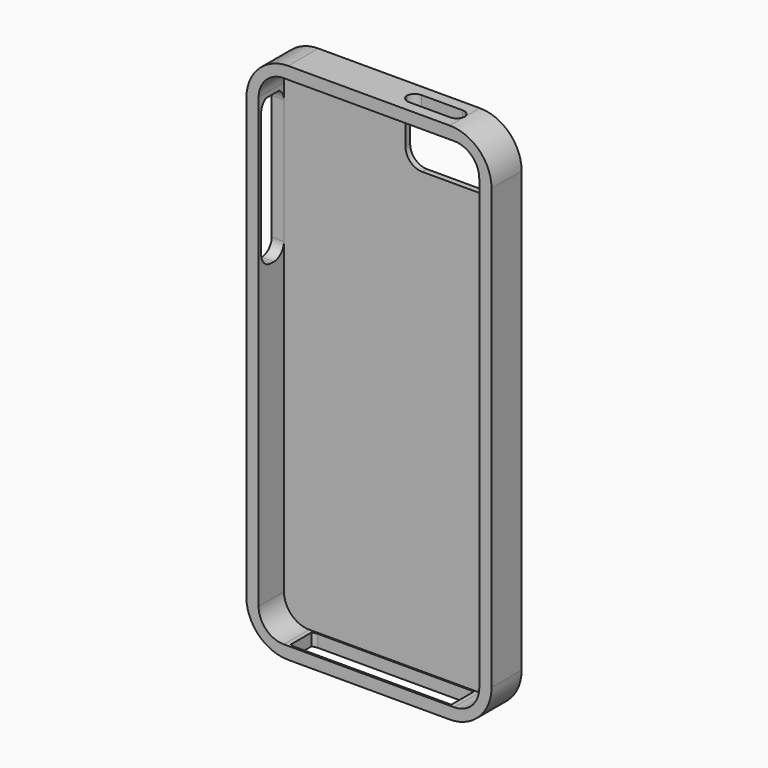
from build123d import *

# Parameters (mm, degrees)
F1_DEPTH      = 9
F3_DEPTH      = 5
F5_DEPTH      = 5.53
F7_DEPTH      = 7.6
F9_DEPTH      = 3
F11_DEPTH     = 25
F12_DEPTH     = 25
F14_DEPTH     = 8
F15_T         = 2.5
F15_T3_DEPTH  = 7.928932
F15_T5_DEPTH  = 13
F15_T7_DEPTH  = 45.742136
F15_T9_DEPTH  = 112.142136
F15_T11_DEPTH = 7.928932
F15_T13_DEPTH = 7.928932
F15_T16_ANGLE = 90
F15_T18_ANGLE = 90
F15_T20_ANGLE = 90
F15_T22_ANGLE = 90


# Not quite as in the source:
# - a shell that OpenCascade refuses in one call is made with other operations: the cavity is built on its own and cut out


with BuildPart() as f1:
    # F0 (on Front) → F1 (new body)
    with BuildSketch(Plane.XZ):
        with BuildLine():
            Line((13.970302, 55.774098), (-24.629698, 55.774098))
            ThreePointArc((-24.629698, 55.774098), (-31.700766, 52.845166), (-34.629698, 45.774098))
            Line((-34.629698, 45.774098), (-34.629698, -59.225902))
            ThreePointArc((-34.629698, -59.225902), (-31.700766, -66.29697), (-24.629698, -69.225902))
            Line((-24.629698, -69.225902), (13.970302, -69.225902))
            ThreePointArc((13.970302, -69.225902), (21.04137, -66.29697), (23.970302, -59.225902))
            Line((23.970302, -59.225902), (23.970302, 45.774098))
            ThreePointArc((23.970302, 45.774098), (21.04137, 52.845166), (13.970302, 55.774098))
        make_face()
    extrude(amount=F1_DEPTH)

    # F2 (on face) → F3 (cut)
    with BuildSketch(Plane(origin=(-34.629698, 0, 0), x_dir=(0, -1, 0), z_dir=(-1, 0, 0))):
        with BuildLine():
            ThreePointArc((1.445644, 13.40758), (2.324323, 11.28626), (4.445644, 10.40758))
            Line((4.445644, 10.40758), (5.235644, 10.40758))
            ThreePointArc((5.235644, 10.40758), (7.356964, 11.28626), (8.235644, 13.40758))
            Line((8.235644, 13.40758), (8.235644, 43.24758))
            ThreePointArc((8.235644, 43.24758), (7.867456, 44.687568), (6.853267, 45.774098))
            Line((6.853267, 45.774098), (2.82802, 45.774098))
            ThreePointArc((2.82802, 45.774098), (1.813831, 44.687568), (1.445644, 43.24758))
            Line((1.445644, 43.24758), (1.445644, 13.40758))
        make_face()
    extrude(amount=-F3_DEPTH, mode=Mode.SUBTRACT)

    # F4 (on face) → F5 (cut)
    with BuildSketch(Plane(origin=(0, 0, -69.225902), x_dir=(1, 0, 0), z_dir=(0, 0, -1))):
        with BuildLine():
            Line((13.596659, 8.527939), (-23.283341, 8.527939))
            ThreePointArc((-23.283341, 8.527939), (-23.975167, 8.447079), (-24.629698, 8.208858))
            Line((-24.629698, 8.208858), (-24.629698, 2.057021))
            ThreePointArc((-24.629698, 2.057021), (-23.975167, 1.818799), (-23.283341, 1.737939))
            Line((-23.283341, 1.737939), (13.596659, 1.737939))
            ThreePointArc((13.596659, 1.737939), (13.783845, 1.743785), (13.970302, 1.761298))
            Line((13.970302, 1.761298), (13.970302, 8.50458))
            ThreePointArc((13.970302, 8.50458), (13.783845, 8.522094), (13.596659, 8.527939))
        make_face()
    extrude(amount=-F5_DEPTH, mode=Mode.SUBTRACT)

    # F6 (on face) → F7 (cut)
    with BuildSketch(Plane.XZ.offset(9)):
        with BuildLine():
            Line((15.04137, 52.845166), (-25.700766, 52.845166))
            ThreePointArc((-25.700766, 52.845166), (-29.943407, 51.087807), (-31.700766, 46.845166))
            Line((-31.700766, 46.845166), (-31.700766, -60.29697))
            ThreePointArc((-31.700766, -60.29697), (-29.943407, -64.53961), (-25.700766, -66.29697))
            Line((-25.700766, -66.29697), (15.04137, -66.29697))
            ThreePointArc((15.04137, -66.29697), (19.28401, -64.53961), (21.04137, -60.29697))
            Line((21.04137, -60.29697), (21.04137, 46.845166))
            ThreePointArc((21.04137, 46.845166), (19.28401, 51.087807), (15.04137, 52.845166))
        make_face()
    extrude(amount=-F7_DEPTH, mode=Mode.SUBTRACT)

    # F8 (on face) → F9 (cut)
    with BuildSketch(Plane.XY.offset(55.774098)):
        with BuildLine():
            Line((2.150302, -6.363066), (11.970302, -6.363066))
            ThreePointArc((11.970302, -6.363066), (13.328609, -5.831058), (13.964286, -4.518066))
            ThreePointArc((13.964286, -4.518066), (13.328609, -3.205074), (11.970302, -2.673066))
            Line((11.970302, -2.673066), (2.150302, -2.673066))
            ThreePointArc((2.150302, -2.673066), (0.791994, -3.205074), (0.156317, -4.518066))
            ThreePointArc((0.156317, -4.518066), (0.791994, -5.831058), (2.150302, -6.363066))
        make_face()
    extrude(amount=-F9_DEPTH, mode=Mode.SUBTRACT)

    # F10 (on face) → F11 (cut)
    with BuildSketch(Plane(origin=(0, 0, 0), x_dir=(-1, 0, 0), z_dir=(0, 1, 0))):
        with BuildLine():
            Line((-1.330302, 51.964098), (-14.630302, 51.964098))
            ThreePointArc((-14.630302, 51.964098), (-17.458729, 50.792525), (-18.630302, 47.964098))
            Line((-18.630302, 47.964098), (-18.630302, 42.834098))
            ThreePointArc((-18.630302, 42.834098), (-17.458729, 40.005671), (-14.630302, 38.834098))
            Line((-14.630302, 38.834098), (-1.330302, 38.834098))
            ThreePointArc((-1.330302, 38.834098), (1.498125, 40.005671), (2.669698, 42.834098))
            Line((2.669698, 42.834098), (2.669698, 47.964098))
            ThreePointArc((2.669698, 47.964098), (1.498125, 50.792525), (-1.330302, 51.964098))
        make_face()
    extrude(amount=-F11_DEPTH, mode=Mode.SUBTRACT)

    # F4 (on face) → F12 (cut)
    with BuildSketch(Plane(origin=(0, 0, -69.225902), x_dir=(1, 0, 0), z_dir=(0, 0, -1))):
        with BuildLine():
            Line((13.596659, 8.527939), (-23.283341, 8.527939))
            ThreePointArc((-23.283341, 8.527939), (-23.975167, 8.447079), (-24.629698, 8.208858))
            Line((-24.629698, 8.208858), (-24.629698, 2.057021))
            ThreePointArc((-24.629698, 2.057021), (-23.975167, 1.818799), (-23.283341, 1.737939))
            Line((-23.283341, 1.737939), (13.596659, 1.737939))
            ThreePointArc((13.596659, 1.737939), (13.783845, 1.743785), (13.970302, 1.761298))
            Line((13.970302, 1.761298), (13.970302, 8.50458))
            ThreePointArc((13.970302, 8.50458), (13.783845, 8.522094), (13.596659, 8.527939))
        make_face()
    extrude(amount=-F12_DEPTH, mode=Mode.SUBTRACT)

    # F13 (on face) → F14 (join)
    with BuildSketch(Plane(origin=(0, 0, 0), x_dir=(-1, 0, 0), z_dir=(0, 1, 0))):
        Polygon((16.75532, 12.947292), (-7.00677, 12.947292), (-15.132455, 0), (-7.00677, 0), (-15.132455, -13.861218), (-7.00677, -13.861218), (-15.132455, -39.359054), (15.536753, -13.861218), (3.046423, -13.861218), (16.75532, 0), (6.702128, 0), align=None)
    extrude(amount=F14_DEPTH)

    # F15: shell of thickness 2.5, made by hand


with BuildPart() as f15_core1:
    # F15_t2: copy of F1
    add(f1.part)

    # the walls: a layer under each face that stays
    f15_faces = [f15_core1.faces().sort_by_distance(p)[0] for p in [
        (21.04137, -4.5, 52.845166),
        (23.970302, -4.5, -6.725902),
        (-5.329698, -4.5, 55.774098),
        (-32.676365, -9, -65.059235),
        (0.791994, -3.205074, 54.309632),
        (7.060302, -2.673066, 54.309632),
        (13.328609, -3.205074, 54.309632),
        (13.328609, -5.831058, 54.309632),
        (7.060302, -6.363066, 54.309632),
        (0.791994, -5.831058, 54.309632),
        (-34.629698, -4.5, -6.725902),
        (-31.700766, -4.5, -66.29697),
        (-11.728724, 4, 0),
        (-9.900872, 4, -6.930609),
        (-9.291588, 4, -13.861218),
        (-0.202149, 4, -26.610136),
        (11.069612, 4, -26.610136),
        (11.069612, 4, -13.861218),
        (11.069612, 4, -6.930609),
        (11.069612, 4, 0),
        (11.069612, 4, 6.473646),
        (-4.874275, 4, 12.947292),
        (-11.728724, 4, 6.473646),
        (-1.498125, -0.7, 50.792525),
        (-2.669698, -0.7, 45.399098),
        (7.980302, -0.7, 51.964098),
        (-1.498125, -0.7, 40.005671),
        (17.458729, -0.7, 50.792525),
        (7.980302, -0.7, 38.834098),
        (18.630302, -0.7, 45.399098),
        (17.458729, -0.7, 40.005671),
        (19.28401, -5.2, 51.087807),
        (-5.329698, -5.2, 52.845166),
        (-29.943407, -5.2, 51.087807),
        (-31.700766, -5.2, -6.725902),
        (-29.943407, -5.2, -64.53961),
        (-24.342695, -1.653333, -66.29697),
        (19.28401, -5.2, -64.53961),
        (21.04137, -5.2, -6.725902),
        (13.970302, -5.132939, -67.761436),
        (-33.165232, -4.840644, 45.774098),
        (13.783845, -1.743785, -67.761436),
        (-4.843341, -1.737939, -67.761436),
        (-23.975167, -1.818799, -67.761436),
        (-33.165232, -7.867456, 44.687568),
        (-33.165232, -8.235644, 28.32758),
        (-33.165232, -7.356964, 11.28626),
        (-33.165232, -4.840644, 10.40758),
        (-33.165232, -2.324323, 11.28626),
        (-33.165232, -1.445644, 28.32758),
        (-33.165232, -1.813831, 44.687568),
        (-24.629698, -5.132939, -67.761436),
        (-0.811433, 8, -13.205881),
        (-5.329698, -1.4, -6.725902),
        (-23.975167, -8.447079, -67.761436),
        (-4.843341, -8.527939, -67.761436),
        (13.783845, -8.522094, -67.761436),
    ]]
    thicken(f15_faces, amount=-F15_T, mode=Mode.SUBTRACT)

    # F15_s4 → F15_t3 (cut)
    with BuildSketch(Plane.XY.offset(50.345166)):
        Polygon((0.206167, -4.518066), (-2.336164, -4.324316), (-2.351225, -4.518066), (-2.336164, -4.711816), align=None)
        Polygon((13.914437, -4.518066), (16.456767, -4.324316), (16.471828, -4.518066), (16.456767, -4.711816), align=None)
    extrude(amount=F15_T3_DEPTH, mode=Mode.SUBTRACT)

    # F15_s6 → F15_t5 (cut)
    with BuildSketch(Plane.XZ.offset(-10.5)):
        Polygon((-6.721875, 0.009668), (-6.702128, -2.5), (-1.595803, -2.5), (-4.727498, 1.533243), align=None)
        Polygon((-3.064198, -13.853798), (-1.268916, -12.103245), (2.942266, -16.361218), (-3.046423, -16.361218), align=None)
        Polygon((7.030589, -13.878628), (4.624799, -14.620308), (3.586188, -11.361218), (7.00677, -11.361218), align=None)
        Polygon((7.028337, -0.012357), (4.850034, -1.264315), (2.643328, 2.5), (7.00677, 2.5), align=None)
    extrude(amount=F15_T5_DEPTH, mode=Mode.SUBTRACT)

    # F15_s8 → F15_t7 (cut)
    with BuildSketch(Plane.YZ.offset(-28.200766)):
        Polygon((-1.425, 52.820166), (-1.4, 55.345166), (1.1, 55.345166), (1.1, 52.845166), align=None)
        Polygon((-1.425, -66.27197), (-1.4, -68.79697), (1.1, -68.79697), (1.1, -66.29697), align=None)
    extrude(amount=F15_T7_DEPTH, mode=Mode.SUBTRACT)

    # F15_s10 → F15_t9 (cut)
    with BuildSketch(Plane.XY.offset(-62.79697)):
        Polygon((-31.675766, -1.425), (-34.200766, -1.4), (-34.200766, 1.1), (-31.700766, 1.1), align=None)
        Polygon((21.01637, -1.425), (23.54137, -1.4), (23.54137, 1.1), (21.04137, 1.1), align=None)
    extrude(amount=F15_T9_DEPTH, mode=Mode.SUBTRACT)

    # F15_s12 → F15_t11 (cut)
    with BuildSketch(Plane.XY.offset(-71.725902)):
        Polygon((13.942188, -8.479775), (16.470302, -8.50458), (16.470302, -10.710386), (14.281671, -10.985114), align=None)
        Polygon((13.942188, -1.786104), (16.470302, -1.761298), (16.470302, 0.444508), (14.281671, 0.719236), align=None)
        Polygon((-24.593479, -2.079362), (-25.751662, 0.177078), (-27.129698, -0.514972), (-27.129698, -2.057021), align=None)
        Polygon((-24.593479, -8.186517), (-27.129698, -8.208858), (-27.129698, -9.750907), (-25.751662, -10.442956), align=None)
    extrude(amount=F15_T11_DEPTH, mode=Mode.SUBTRACT)

    # F15_s14 → F15_t13 (cut)
    with BuildSketch(Plane.YZ.offset(-37.129698)):
        Polygon((-2.8415, 45.728044), (-2.82802, 48.274098), (-2.096265, 48.274098), (-1.480001, 47.87953), align=None)
        Polygon((-6.839787, 45.728044), (-6.853267, 48.274098), (-7.585022, 48.274098), (-8.201287, 47.87953), align=None)
    extrude(amount=F15_T13_DEPTH, mode=Mode.SUBTRACT)

    # F15_s15 → F15_t16 (revolve, cut)
    with BuildSketch(Plane.XY.offset(46.845166)):
        Polygon((21.01637, -1.425), (23.54137, -1.4), (23.54137, 1.1), (21.04137, 1.1), align=None)
    revolve(axis=Axis((15.04137, -1.4, 46.845166), (0, -1, 0)), revolution_arc=F15_T16_ANGLE, mode=Mode.SUBTRACT)

    # F15_s17 → F15_t18 (revolve, cut)
    with BuildSketch(Plane.YZ.offset(-25.700766)):
        Polygon((-1.425, 52.820166), (-1.4, 55.345166), (1.1, 55.345166), (1.1, 52.845166), align=None)
    revolve(axis=Axis((-25.700766, -1.4, 46.845166), (0, -1, 0)), revolution_arc=F15_T18_ANGLE, mode=Mode.SUBTRACT)

    # F15_s19 → F15_t20 (revolve, cut)
    with BuildSketch(Plane.XY.offset(-60.29697)):
        Polygon((-31.675766, -1.425), (-34.200766, -1.4), (-34.200766, 1.1), (-31.700766, 1.1), align=None)
    revolve(axis=Axis((-25.700766, -1.4, -60.29697), (0, -1, 0)), revolution_arc=F15_T20_ANGLE, mode=Mode.SUBTRACT)

    # F15_s21 → F15_t22 (revolve, cut)
    with BuildSketch(Plane.YZ.offset(15.04137)):
        Polygon((-1.425, -66.27197), (-1.4, -68.79697), (1.1, -68.79697), (1.1, -66.29697), align=None)
    revolve(axis=Axis((15.04137, -1.4, -60.29697), (0, -1, 0)), revolution_arc=F15_T22_ANGLE, mode=Mode.SUBTRACT)


with BuildPart() as f1_1:
    add(f1.part)

    # what is left inside the walls is the cavity
    f15_cavity = [f15_core1.part.solids().sort_by_distance(p)[0] for p in [
        (18.351784, -4.333333, -68.187109),
        (-0.439991, 5.475, -17.829776),
    ]]
    add(f15_cavity, mode=Mode.SUBTRACT)


solid = f1_1.part
